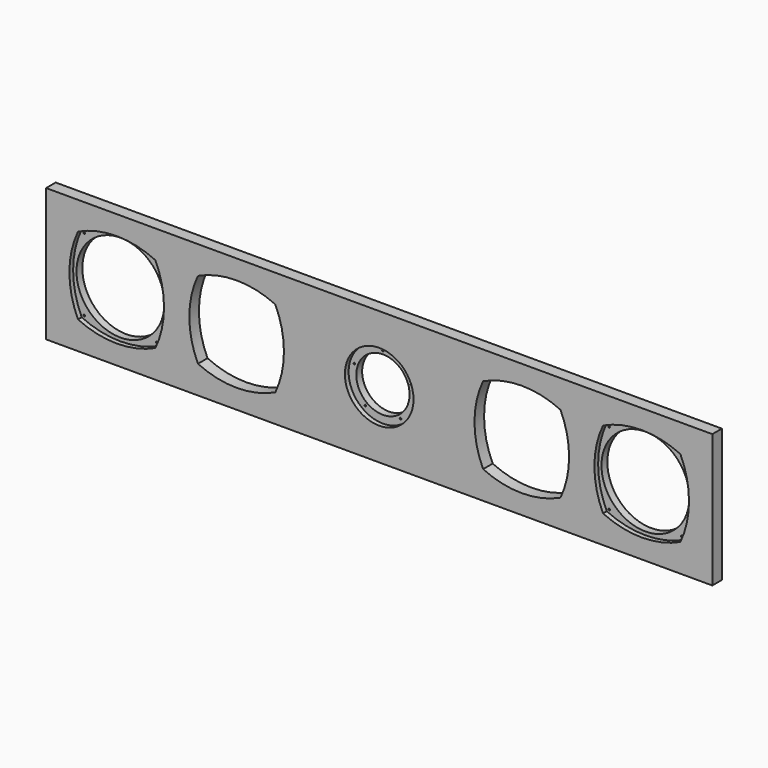
from build123d import *

# Parameters (mm, degrees)
F0_W     = 1000
F0_H     = 200
F0_R     = 51.5
F1_DEPTH = 18
F0_R_2   = 1.25
F0_R_3   = 66
F0_R_4   = 40
F2_DEPTH = 11


# Not quite as in the source:
# - a feature names something its author has since deleted; it is built from what else it names


with BuildPart() as f1:
    # F0 (on Front) → F1 (new body)
    with BuildSketch(Plane.XZ):
        Rectangle(F0_W, F0_H)
        with BuildLine():
            ThreePointArc((-452.0796354846, 58.0796354846), (-394, 71), (-335.9203645154, 58.0796354846))
            ThreePointArc((-335.9203645154, 58.0796354846), (-323, 0), (-335.9203645154, -58.0796354846))
            ThreePointArc((-335.9203645154, -58.0796354846), (-394, -71), (-452.0796354846, -58.0796354846))
            ThreePointArc((-452.0796354846, -58.0796354846), (-465, 0), (-452.0796354846, 58.0796354846))
        make_face(mode=Mode.SUBTRACT)
        with BuildLine():
            ThreePointArc((-272.0796354846, 58.0796354846), (-214, 71), (-155.9203645154, 58.0796354846))
            ThreePointArc((-155.9203645154, 58.0796354846), (-143, 0), (-155.9203645154, -58.0796354846))
            ThreePointArc((-155.9203645154, -58.0796354846), (-214, -71), (-272.0796354846, -58.0796354846))
            ThreePointArc((-272.0796354846, -58.0796354846), (-285, 0), (-272.0796354846, 58.0796354846))
        make_face(mode=Mode.SUBTRACT)
        Circle(F0_R, mode=Mode.SUBTRACT)
        with BuildLine():
            ThreePointArc((155.9203645154, -58.0796354846), (143, 0), (155.9203645154, 58.0796354846))
            ThreePointArc((155.9203645154, 58.0796354846), (214, 71), (272.0796354846, 58.0796354846))
            ThreePointArc((272.0796354846, 58.0796354846), (285, 0), (272.0796354846, -58.0796354846))
            ThreePointArc((272.0796354846, -58.0796354846), (214, -71), (155.9203645154, -58.0796354846))
        make_face(mode=Mode.SUBTRACT)
        with BuildLine():
            ThreePointArc((335.9203645154, 58.0796354846), (394, 71), (452.0796354846, 58.0796354846))
            ThreePointArc((452.0796354846, 58.0796354846), (465, 0), (452.0796354846, -58.0796354846))
            ThreePointArc((452.0796354846, -58.0796354846), (394, -71), (335.9203645154, -58.0796354846))
            ThreePointArc((335.9203645154, -58.0796354846), (323, 0), (335.9203645154, 58.0796354846))
        make_face(mode=Mode.SUBTRACT)
    extrude(amount=F1_DEPTH)

    # F0 (on Front) → F2 (join)
    with BuildSketch(Plane.XZ):
        with BuildLine():
            ThreePointArc((-335.9203645154, -58.0796354846), (-323, 0), (-335.9203645154, 58.0796354846))
            ThreePointArc((-335.9203645154, 58.0796354846), (-394, 71), (-452.0796354846, 58.0796354846))
            ThreePointArc((-452.0796354846, 58.0796354846), (-465, 0), (-452.0796354846, -58.0796354846))
            ThreePointArc((-452.0796354846, -58.0796354846), (-394, -71), (-335.9203645154, -58.0796354846))
        make_face()
        with Locations((-448.5441015786, -54.5441015786)):
            Circle(F0_R_2, mode=Mode.SUBTRACT)
        with Locations((-339.4558984214, -54.5441015786)):
            Circle(F0_R_2, mode=Mode.SUBTRACT)
        with Locations((-394, 0)):
            Circle(F0_R_3, mode=Mode.SUBTRACT)
        with Locations((-448.5441015786, 54.5441015786)):
            Circle(F0_R_2, mode=Mode.SUBTRACT)
        with Locations((-339.4558984214, 54.5441015786)):
            Circle(F0_R_2, mode=Mode.SUBTRACT)
        with BuildLine():
            ThreePointArc((452.0796354846, -58.0796354846), (465, 0), (452.0796354846, 58.0796354846))
            ThreePointArc((452.0796354846, 58.0796354846), (394, 71), (335.9203645154, 58.0796354846))
            ThreePointArc((335.9203645154, 58.0796354846), (323, 0), (335.9203645154, -58.0796354846))
            ThreePointArc((335.9203645154, -58.0796354846), (394, -71), (452.0796354846, -58.0796354846))
        make_face()
        with Locations((339.4558984214, -54.5441015786)):
            Circle(F0_R_2, mode=Mode.SUBTRACT)
        with Locations((448.5441015786, -54.5441015786)):
            Circle(F0_R_2, mode=Mode.SUBTRACT)
        with Locations((394, 0)):
            Circle(F0_R_3, mode=Mode.SUBTRACT)
        with Locations((339.4558984214, 54.5441015786)):
            Circle(F0_R_2, mode=Mode.SUBTRACT)
        with Locations((448.5441015786, 54.5441015786)):
            Circle(F0_R_2, mode=Mode.SUBTRACT)
        Circle(F0_R)
        with BuildLine():
            ThreePointArc((43.1672658205, 12.7116938911), (44.5394598189, 6.4215667122), (45, 0))
            ThreePointArc((45, 0), (40.3751702485, -19.8707228708), (27.4513054486, -35.6570586163))
            ThreePointArc((27.4513054486, -35.6570586163), (27.6364458273, -36.0112469205), (27.7003363532, -36.4057647469))
            ThreePointArc((27.7003363532, -36.4057647469), (26.8283423835, -37.5972392288), (25.4289580476, -37.1263800096))
            ThreePointArc((25.4289580476, -37.1263800096), (0, -45), (-25.4289580476, -37.1263800096))
            ThreePointArc((-25.4289580476, -37.1263800096), (-27.1850679185, -37.4170359898), (-27.4513054486, -35.6570586163))
            ThreePointArc((-27.4513054486, -35.6570586163), (-42.7975432333, -13.9057647469), (-43.1672658205, 12.7116938911))
            ThreePointArc((-43.1672658205, 12.7116938911), (-43.9863638787, 14.2920359898), (-42.3947978504, 15.0891058459))
            ThreePointArc((-42.3947978504, 15.0891058459), (-26.4503363532, 36.4057647469), (-1.2498794309, 44.9826388889))
            ThreePointArc((-1.2498794309, 44.9826388889), (-0.0086807649, 46.2499698574), (1.25, 45))
            ThreePointArc((1.25, 45), (1.2499698574, 44.9913192351), (1.2498794309, 44.9826388889))
            ThreePointArc((1.2498794309, 44.9826388889), (26.4503363532, 36.4057647469), (42.3947978504, 15.0891058459))
            ThreePointArc((42.3947978504, 15.0891058459), (43.5252341949, 14.9221140295), (44.0475432333, 13.9057647469))
            ThreePointArc((44.0475432333, 13.9057647469), (43.8036876648, 13.1640280126), (43.1672658205, 12.7116938911))
        make_face(mode=Mode.SUBTRACT)
        with BuildLine():
            ThreePointArc((27.4513054486, -35.6570586163), (40.3751702485, -19.8707228708), (45, 0))
            ThreePointArc((45, 0), (44.5394598189, 6.4215667122), (43.1672658205, 12.7116938911))
            ThreePointArc((43.1672658205, 12.7116938911), (41.6087225879, 13.5194935039), (42.3947978504, 15.0891058459))
            ThreePointArc((42.3947978504, 15.0891058459), (26.4503363532, 36.4057647469), (1.2498794309, 44.9826388889))
            ThreePointArc((1.2498794309, 44.9826388889), (0, 43.75), (-1.2498794309, 44.9826388889))
            ThreePointArc((-1.2498794309, 44.9826388889), (-26.4503363532, 36.4057647469), (-42.3947978504, 15.0891058459))
            ThreePointArc((-42.3947978504, 15.0891058459), (-41.7811939506, 14.6334557085), (-41.5475432333, 13.9057647469))
            ThreePointArc((-41.5475432333, 13.9057647469), (-42.055806499, 12.8996203154), (-43.1672658205, 12.7116938911))
            ThreePointArc((-43.1672658205, 12.7116938911), (-42.7975432333, -13.9057647469), (-27.4513054486, -35.6570586163))
            ThreePointArc((-27.4513054486, -35.6570586163), (-26.0558185268, -35.2196552727), (-25.2003363532, -36.4057647469))
            ThreePointArc((-25.2003363532, -36.4057647469), (-25.2588618713, -36.7837707772), (-25.4289580476, -37.1263800096))
            ThreePointArc((-25.4289580476, -37.1263800096), (0, -45), (25.4289580476, -37.1263800096))
            ThreePointArc((25.4289580476, -37.1263800096), (25.7156047878, -35.3944935039), (27.4513054486, -35.6570586163))
        make_face()
        Circle(F0_R_4, mode=Mode.SUBTRACT)
    extrude(amount=F2_DEPTH)


solid = f1.part
